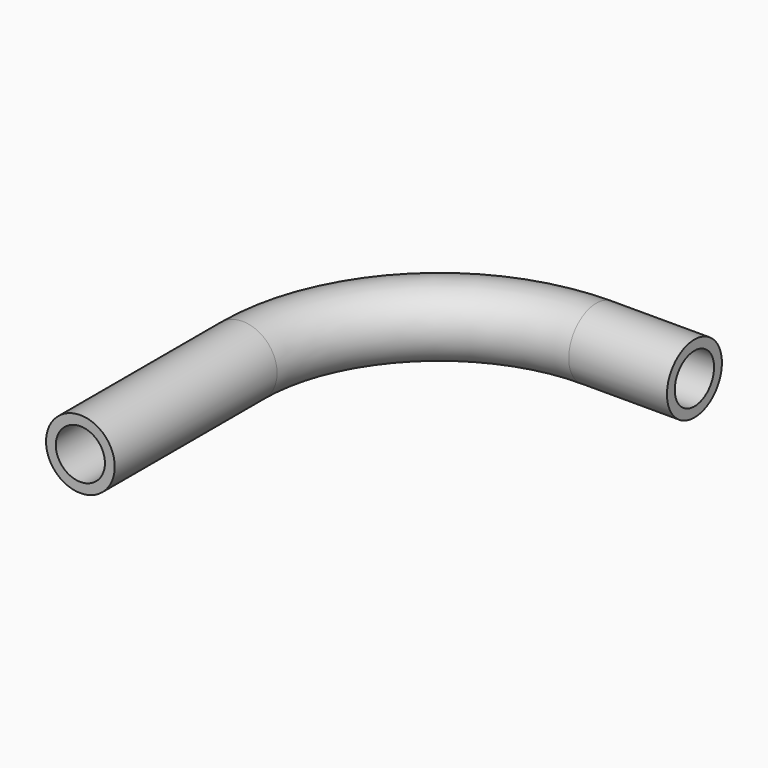
from build123d import *
from build123d import SkipClean  # not in build123d's __all__

# Parameters (mm, degrees)
F0_W        = 1.5
F0_H        = 15
F0_W_2      = 15
F0_H_2      = 1.5
F1_FACE_R   = 5.25
F1_FACE_R_2 = 3.75
F3_FACE_R   = 5.25
F3_FACE_R_2 = 3.75
F6_R        = 5.25
F6_R_2      = 3.75
F6_R_3      = 2.5
F7_DEPTH    = 1
F8_R        = 5.25
F8_R_2      = 3.75
F9_DEPTH    = 15


# Not quite as in the source:
# - after a boolean that leaves OpenCascade's solid faulty, fix() repairs it


with BuildPart() as f1:
    # F0 (on Top) → F1 (revolve)
    with BuildSketch(Plane.XY):
        with Locations((-34.5, -7.5)):
            Rectangle(F0_W, F0_H)
        with Locations((-25.5, -7.5)):
            Rectangle(F0_W, F0_H)
    revolve(axis=Axis((-30, -7.5, 0), (0, -1, 0)))



with BuildPart() as f3:
    # F0 (on Top) → F3 (revolve)
    with BuildSketch(Plane.XY):
        with Locations((7.5, 25.5)):
            Rectangle(F0_W_2, F0_H_2)
        with Locations((7.5, 34.5)):
            Rectangle(F0_W_2, F0_H_2)
    revolve(axis=Axis((16.0269476473, 30, 0), (1, 0, 0)))


with BuildPart() as f1_1:
    add(f1.part, clean=False)

    add(f3.part)  # F5 merges F3
    # F5: sweep along a path in F4
    with BuildLine(Plane.XY) as f5_path:
        ThreePointArc((-30, 0), (-21.2132034356, 21.2132034356), (0, 30))
    # F1_face (on face) + F3_face (on face) → F5 (sweep)
    with BuildSketch(Plane(origin=(-30, 0, 0), x_dir=(-1, 0, 0), z_dir=(0, 1, 0))):
        Circle(F1_FACE_R)
        Circle(F1_FACE_R_2, mode=Mode.SUBTRACT)
    with BuildSketch(Plane(origin=(0, 30, 0), x_dir=(0, -1, 0), z_dir=(-1, 0, 0))):
        Circle(F3_FACE_R)
        Circle(F3_FACE_R_2, mode=Mode.SUBTRACT)
    sweep(path=f5_path.line)

    # F6 (on face) → F7 (join)
    with BuildSketch(Plane.XZ.offset(15)):
        with Locations((-30, 0)):
            Circle(F6_R)
        with Locations((-30, 0)):
            Circle(F6_R_2, mode=Mode.SUBTRACT)
        with Locations((-30, 0)):
            Circle(F6_R_2)
        with Locations((-30, 0)):
            Circle(F6_R_3, mode=Mode.SUBTRACT)
    with SkipClean():  # cleaning this boolean's faces spoils the solid; the shape is the same uncleaned
        extrude(amount=F7_DEPTH)

    # F8 (on face) → F9 (join)
    with BuildSketch(Plane.XZ.offset(16)):
        with Locations((-30, 0)):
            Circle(F8_R)
        with Locations((-30, 0)):
            Circle(F8_R_2, mode=Mode.SUBTRACT)
    extrude(amount=F9_DEPTH)

    add(f1_1.part.fix(), mode=Mode.REPLACE)


solid = f1_1.part
